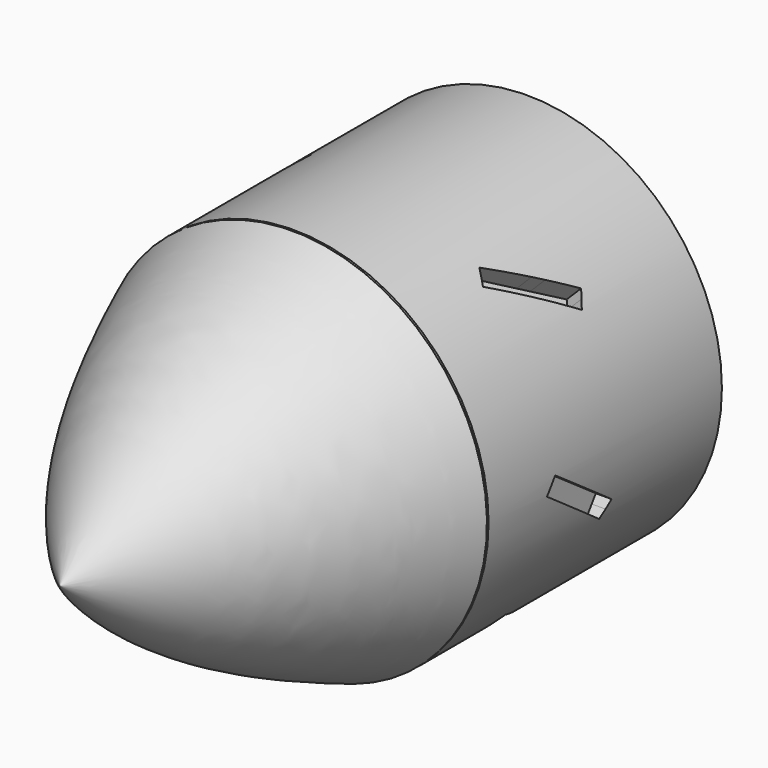
from build123d import *

# Parameters (mm, degrees)
F0_R      = 25.4
F1_DEPTH  = 38.1
F21_DEPTH = 2.794
F22_DEPTH = 2.794
F23_DEPTH = 2.794
F24_DEPTH = 2.794
F25_DEPTH = 2.794
F26_DEPTH = 2.794
F27_DEPTH = 2.794


with BuildPart() as f1:
    # F0 (on Front) → F1 (new body)
    with BuildSketch(Plane.XZ):
        Circle(F0_R)
    extrude(amount=F1_DEPTH)

    # F14 (on face) → F21 (cut)
    with BuildSketch(Plane(origin=(17.9605122421, 0, 17.9605122421), x_dir=(0, 1, 0), z_dir=(0.7071067812, 0, 0.7071067812))):
        Polygon((-22.2601667082, -0.9570972485), (-17.2041964605, -4.497325729), (-16.5340297522, -3.5402284804), (-21.59, 0), align=None)
        Polygon((-27.316136956, 2.5831312319), (-22.2601667082, -0.9570972485), (-21.59, 0), (-20.9198332918, 0.9570972485), (-25.9758035395, 4.497325729), align=None)
        Polygon((-21.59, 0), (-16.5340297522, -3.5402284804), (-15.863863044, -2.5831312319), (-19.552956764, 0), align=None)
        Polygon((-20.9198332918, 0.9570972485), (-21.59, 0), (-19.552956764, 0), align=None)
    extrude(amount=-F21_DEPTH, mode=Mode.SUBTRACT)

    # F20 (on offset) → F22 (cut)
    with BuildSketch(Plane.YZ.offset(25.4)):
        Polygon((-28.5544317948, -0.9064046195), (-18.4424912993, -7.9868615804), (-17.772324591, -7.0297643319), (-22.8282948388, -3.4895358514), (-21.4186995436, -3.4895358514), (-20.7912516028, -3.4895358514), (-27.2140983783, 1.0077898775), align=None)
        Polygon((-22.8282948388, -3.4895358514), (-17.772324591, -7.0297643319), (-17.1021578828, -6.0726670833), (-20.7912516028, -3.4895358514), (-21.4186995436, -3.4895358514), align=None)
    extrude(amount=-F22_DEPTH, mode=Mode.SUBTRACT)

    # F19 (on face) → F23 (cut)
    with BuildSketch(Plane(origin=(17.9605122421, 0, -17.9605122421), x_dir=(0, 1, 0), z_dir=(0.7071067812, 0, -0.7071067812))):
        Polygon((-27.8651035773, -1.3890774337), (-17.7531630818, -8.4695343946), (-17.0829963736, -7.5124371461), (-22.1389666213, -3.9722086656), (-20.1019233853, -3.9722086656), (-26.5247701609, 0.5251170634), align=None)
        Polygon((-22.1389666213, -3.9722086656), (-17.0829963736, -7.5124371461), (-16.4128296653, -6.5553398975), (-20.1019233853, -3.9722086656), align=None)
    extrude(amount=-F23_DEPTH, mode=Mode.SUBTRACT)

    # F18 (on offset) → F24 (cut)
    with BuildSketch(Plane.XY.offset(-25.4)):
        Polygon((-6.3771515661, -16.7774689451), (0.7033053948, -26.8894094406), (2.6174998919, -25.5490760241), (-1.8798258371, -19.1262292486), (-1.8798258371, -21.1632724846), (-5.4200543175, -16.1073022368), align=None)
        Polygon((-4.462957069, -15.4371355286), (-5.4200543175, -16.1073022368), (-1.8798258371, -21.1632724846), (-1.8798258371, -19.1262292486), align=None)
    extrude(amount=F24_DEPTH, mode=Mode.SUBTRACT)

    # F17 (on face) → F25 (cut)
    with BuildSketch(Plane(origin=(-17.9605122421, 0, -17.9605122421), x_dir=(0, 1, 0), z_dir=(0.7071067812, 0, 0.7071067812))):
        Polygon((-20.5471214297, 3.5909211094), (-16.8580277097, 6.1740523413), (-17.5281944179, 7.1311495899), (-22.5841646657, 3.5909211094), align=None)
        Polygon((-26.9699682052, -0.9064046195), (-20.5471214297, 3.5909211094), (-22.5841646657, 3.5909211094), (-17.5281944179, 7.1311495899), (-18.1983611261, 8.0882468384), (-28.3103016217, 1.0077898775), align=None)
    extrude(amount=F25_DEPTH, mode=Mode.SUBTRACT)

    # F16 (on offset) → F26 (cut)
    with BuildSketch(Plane.YZ.offset(-25.4)):
        Polygon((-20.6038281526, 3.6719067028), (-16.9147344326, 6.2550379347), (-17.5849011408, 7.2121351832), (-22.6408713886, 3.6719067028), align=None)
        Polygon((-27.0266749281, -0.8254190262), (-20.6038281526, 3.6719067028), (-22.6408713886, 3.6719067028), (-17.5849011408, 7.2121351832), (-18.2550678491, 8.1692324318), (-28.3670083446, 1.0887754709), align=None)
    extrude(amount=F26_DEPTH, mode=Mode.SUBTRACT)

    # F15 (on face) → F27 (cut)
    with BuildSketch(Plane(origin=(-17.9605122421, 0, 17.9605122421), x_dir=(0, 1, 0), z_dir=(0.7071067812, 0, -0.7071067812))):
        Polygon((-21.59, 0), (-20.9198332918, -0.9570972485), (-19.552956764, 0), align=None)
        Polygon((-25.9758035395, -4.497325729), (-20.9198332918, -0.9570972485), (-21.59, 0), (-22.2601667082, 0.9570972485), (-27.316136956, -2.5831312319), align=None)
        Polygon((-21.59, 0), (-19.552956764, 0), (-15.863863044, 2.5831312319), (-16.5340297522, 3.5402284804), align=None)
        Polygon((-22.2601667082, 0.9570972485), (-21.59, 0), (-16.5340297522, 3.5402284804), (-17.2041964605, 4.497325729), align=None)
    extrude(amount=F27_DEPTH, mode=Mode.SUBTRACT)


with BuildPart() as f3:
    # F2 (on Right) → F3 (revolve)
    with BuildSketch(Plane.YZ):
        with BuildLine():
            Line((-38.3663102984, 0), (-76.3406405559, 0))
            add(Edge.make_bspline(
                [(-38.3663102984, -25.4), (-54.5826740563, -18.9965814352), (-65.9471228719, -12.1034290642), (-76.3406405559, 0)],
                knots=[0, 0, 0, 0, 45.6859908342, 45.6859908342, 45.6859908342, 45.6859908342], degree=3))
            Line((-38.3663102984, -25.4), (-38.3663102984, 0))
        make_face()
    revolve(axis=Axis((0, -57.3534754272, 0), (0, 1, 0)))


solid = Compound([f1.part, f3.part])
